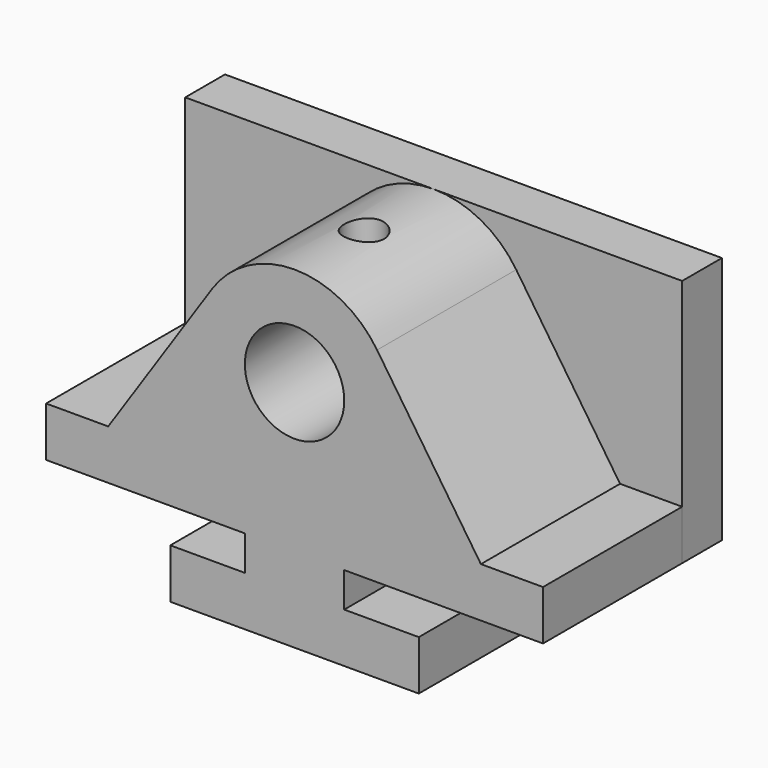
from build123d import *

# Parameters (mm, degrees)
F0_R     = 12.7
F1_DEPTH = 44.45
F3_DEPTH = 12.7
F5_START = 63.5
F4_R     = 5.08
F5_DEPTH = 21.591


# Not quite as in the source:
# - ends of sketch curves that miss each other by under 0.0002 mm in the source are joined


with BuildPart() as f1:
    # F0 (on Front) → F1 (new body)
    with BuildSketch(Plane.XZ):
        with BuildLine():
            Line((0, 0), (31.75, 0))
            Line((31.75, 0), (31.7500008563, 12.7))
            Line((31.7500008563, 12.7), (12.7000008563, 12.7))
            Line((12.7000008563, 12.7), (12.7000008563, 21.59))
            Line((12.7000008563, 21.59), (63.5000008563, 21.59))
            Line((63.5000008563, 21.59), (63.5000008563, 34.29))
            Line((63.5000008563, 34.29), (47.6250008563, 34.29))
            Line((47.6250008563, 34.29), (21.0934264618, 73.8401730104))
            ThreePointArc((21.0934264618, 73.8401730104), (8.563e-07, 85.09), (-21.0934247492, 73.8401730104))
            Line((-21.0934247492, 73.8401730104), (-47.6249991437, 34.29))
            Line((-47.6249991437, 34.29), (-63.4999991437, 34.29))
            Line((-63.4999991437, 34.29), (-63.4999991437, 21.59))
            Line((-63.4999991437, 21.59), (-12.6999991437, 21.59))
            Line((-12.6999991437, 21.59), (-12.6999991437, 12.7))
            Line((-12.6999991437, 12.7), (-31.7499991437, 12.7))
            Line((-31.7499991437, 12.7), (-31.7499991437, 0))
            Line((-31.7499991437, 0), (0, 0))
        make_face()
        with Locations((8.563e-07, 59.69)):
            Circle(F0_R, mode=Mode.SUBTRACT)
    extrude(amount=F1_DEPTH)

    # F2 (on face) → F3 (join)
    with BuildSketch(Plane(origin=(0, 0, 0), x_dir=(-1, 0, 0), z_dir=(0, 1, 0))):
        with BuildLine():
            Line((-63.5, 85.09), (-63.500000685, 34.29))
            Line((-63.500000685, 34.29), (-47.6250008563, 34.29))
            Line((-47.6250008563, 34.29), (-21.0934264618, 73.8401730104))
            ThreePointArc((-21.0934264618, 73.8401730104), (-11.9529420328, 82.1017647059), (-8.563e-07, 85.09))
            Line((-8.563e-07, 85.09), (-63.5, 85.09))
        make_face()
        Polygon((-63.5000008563, 21.59), (0, 21.59), (63.5, 21.59), (63.5, 85.09), (-63.5, 85.09), align=None)
    extrude(amount=F3_DEPTH)

    # F4 (on Top) → F5 (cut)
    with BuildSketch(Plane.XY.offset(F5_START)):
        with Locations((0, -22.225)):
            Circle(F4_R)
    extrude(amount=F5_DEPTH, mode=Mode.SUBTRACT)


solid = f1.part
